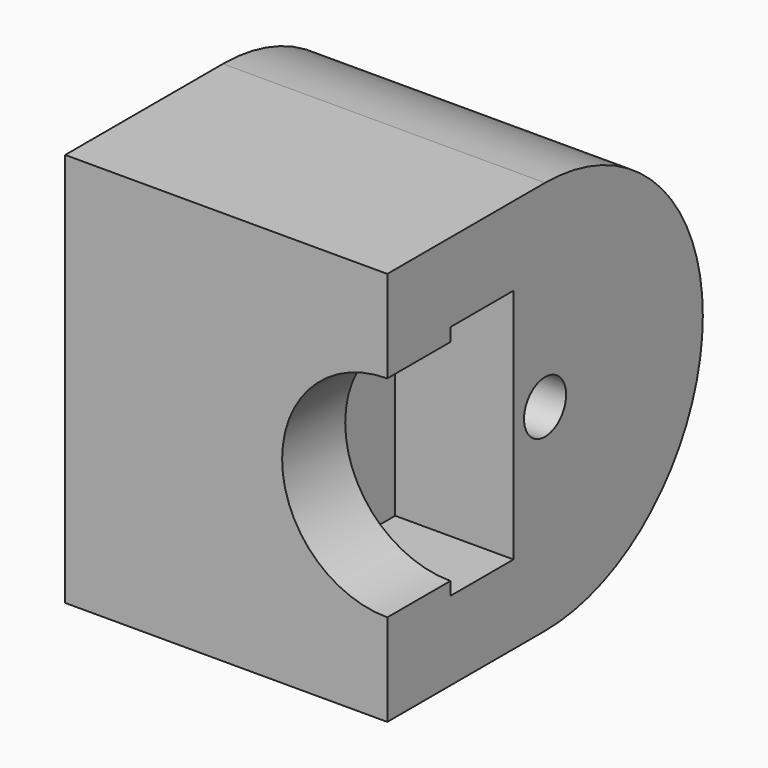
from build123d import *

# Parameters (mm, degrees)
F0_W     = 12.25
F0_H     = 15
F1_DEPTH = 15
F2_R     = 7.49999
F3_R     = 1
F4_DEPTH = 25
F6_DEPTH = 4.5
F8_DEPTH = 3


# Not quite as in the source:
# - a fillet or chamfer is up to 0.001 mm smaller than in the source, because OpenCascade refuses the exact size


with BuildPart() as f1:
    # F0 (on Front) → F1 (new body)
    with BuildSketch(Plane.XZ):
        with Locations((-33.7760131806, 25.872811313)):
            Rectangle(F0_W, F0_H)
    extrude(amount=F1_DEPTH)

    # F2 (radius 7.5 in the source; OpenCascade refuses exactly that, so slightly less here)
    f2_edges = [f1.edges().sort_by_distance(p)[0] for p in [
        (-33.776013, 0, 18.372811),
        (-33.776013, 0, 33.372811),
    ]]
    fillet(f2_edges, radius=F2_R)

    # F3 (on face) → F4 (cut)
    with BuildSketch(Plane(origin=(-39.9010131806, 0, 0), x_dir=(0, -1, 0), z_dir=(-1, 0, 0))):
        with Locations((7.5, 25.872811313)):
            Circle(F3_R)
    extrude(amount=-F4_DEPTH, mode=Mode.SUBTRACT)

    # F5 (on face) → F6 (cut)
    with BuildSketch(Plane.YZ.offset(-27.6510131806)):
        Polygon((-9, 30.372811313), (-15, 30.372811313), (-15, 21.372811313), (-9, 21.372811313), (-9, 25.872811313), align=None)
    extrude(amount=-F6_DEPTH, mode=Mode.SUBTRACT)

    # F7 (on face) → F8 (join)
    with BuildSketch(Plane.XZ.offset(15)):
        with BuildLine():
            Line((-27.6510131806, 30.372811313), (-32.1510131806, 30.372811313))
            Line((-32.1510131806, 30.372811313), (-32.1510131806, 21.372811313))
            Line((-32.1510131806, 21.372811313), (-27.6510131806, 21.372811313))
            Line((-27.6510131806, 21.372811313), (-27.6510131806, 21.872811313))
            ThreePointArc((-27.6510131806, 21.872811313), (-31.6510131806, 25.872811313), (-27.6510131806, 29.872811313))
            Line((-27.6510131806, 29.872811313), (-27.6510131806, 30.372811313))
        make_face()
    extrude(amount=-F8_DEPTH)


solid = f1.part
